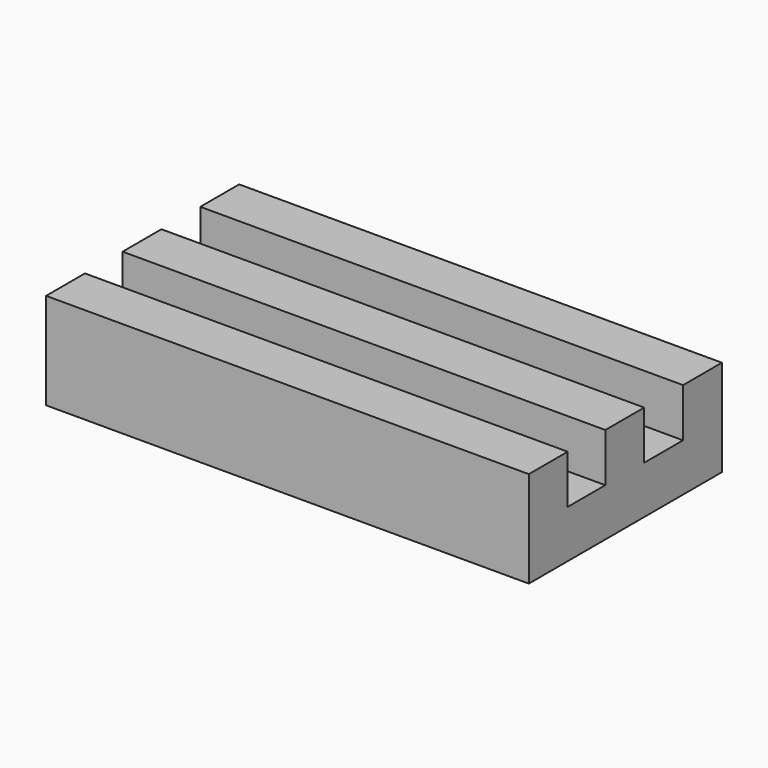
from build123d import *

# Parameters (mm, degrees)
F0_W     = 12.7
F0_H     = 1.6002
F0_H_2   = 1.5494
F0_W_2   = 1.6002
F1_DEPTH = 3.175
F2_T     = -1.6002
F3_DEPTH = 25.4
F4_W     = 12.7
F4_H     = 1.6002
F4_W_2   = 1.6002
F4_H_2   = 1.5494
F5_DEPTH = 1.6002


with BuildPart() as f1:
    # F0 (on Top) → F1 (new body)
    with BuildSketch(Plane.XY):
        with Locations((-5.0789434463, 30.2115620618)):
            Rectangle(F0_W, F0_H)
        with Locations((-5.0789434463, 28.6113620618)):
            Rectangle(F0_W, F0_H)
        with Locations((-5.0789434463, 25.4363620618)):
            Rectangle(F0_W, F0_H_2)
        with Locations((-5.0789434463, 23.8615620618)):
            Rectangle(F0_W, F0_H)
        with Locations((-5.0789434463, 27.0111620618)):
            Rectangle(F0_W, F0_H)
        with Locations((-12.2290434463, 30.2115620618)):
            Rectangle(F0_W_2, F0_H)
        with Locations((-12.2290434463, 27.0111620618)):
            Rectangle(F0_W_2, F0_H)
        with Locations((-12.2290434463, 23.8615620618)):
            Rectangle(F0_W_2, F0_H)
        with Locations((2.0711565537, 30.2115620618)):
            Rectangle(F0_W_2, F0_H)
        with Locations((2.0711565537, 27.0111620618)):
            Rectangle(F0_W_2, F0_H)
        with Locations((2.0711565537, 23.8615620618)):
            Rectangle(F0_W_2, F0_H)
        with Locations((-12.2290434463, 28.6113620618)):
            Rectangle(F0_W_2, F0_H)
        with Locations((-12.2290434463, 25.4363620618)):
            Rectangle(F0_W_2, F0_H_2)
        with Locations((2.0711565537, 28.6113620618)):
            Rectangle(F0_W_2, F0_H)
        with Locations((2.0711565537, 25.4363620618)):
            Rectangle(F0_W_2, F0_H_2)
    extrude(amount=F1_DEPTH)

    # F2
    f2_openings = [f1.faces().sort_by_distance(p)[0] for p in [
        (-5.078943, 27.036562, 0),
    ]]
    offset(amount=F2_T, openings=f2_openings)

    # F0 (on Top) → F3 (cut)
    with BuildSketch(Plane.XY):
        with Locations((-5.0789434463, 25.4363620618)):
            Rectangle(F0_W, F0_H_2)
        with Locations((-5.0789434463, 28.6113620618)):
            Rectangle(F0_W, F0_H)
    extrude(amount=F3_DEPTH, mode=Mode.SUBTRACT)

    # F4 (on face) → F5 (cut)
    with BuildSketch(Plane.XY.offset(3.175)):
        with Locations((-5.0789434463, 28.6113620618)):
            Rectangle(F4_W, F4_H)
        with Locations((2.0711565537, 28.6113620618)):
            Rectangle(F4_W_2, F4_H)
        with Locations((-12.2290434463, 28.6113620618)):
            Rectangle(F4_W_2, F4_H)
        with Locations((2.0711565537, 25.4363620618)):
            Rectangle(F4_W_2, F4_H_2)
        with Locations((-12.2290434463, 25.4363620618)):
            Rectangle(F4_W_2, F4_H_2)
    extrude(amount=-F5_DEPTH, mode=Mode.SUBTRACT)


solid = f1.part
